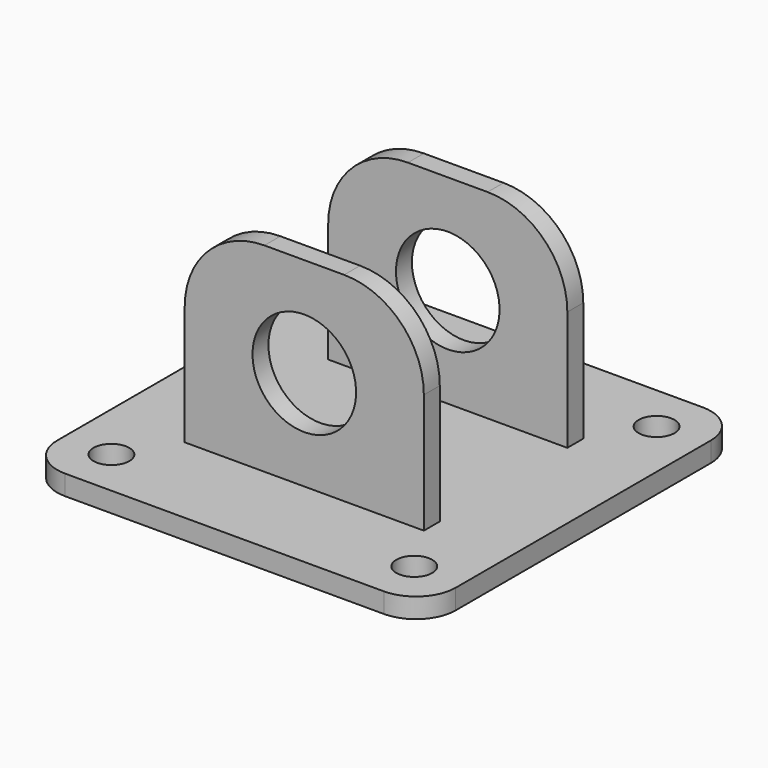
from build123d import *

# Parameters (mm, degrees)
F1_W     = 100
F1_H     = 100
F2_DEPTH = 5
F3_R     = 10
F5_D     = 9
F6_W     = 60
F6_H     = 5
F7_DEPTH = 50
F8_R     = 20
F10_D    = 26


# Not quite as in the source:
# - a pattern or mirror of a feature is missing from the dataset's text; its kind, count and spacing are read off the source's solid


with BuildPart() as f2:
    # F1 (on Top) → F2 (new body)
    with BuildSketch(Plane.XY):
        Rectangle(F1_W, F1_H)
    extrude(amount=F2_DEPTH)

    # F3
    f3_edges = [f2.edges().sort_by_distance(p)[0] for p in [
        (-50, 50, 2.5),
        (-50, -50, 2.5),
        (50, -50, 2.5),
        (50, 50, 2.5),
    ]]
    fillet(f3_edges, radius=F3_R)

    # F5 (through all)
    with Locations(Plane.XY.offset(5)):
        with Locations((-38, -38), (38, -38), (-38, -38), (38, 38)):
            f5 = Hole(F5_D / 2)

    # F5_copies: F5 across plane
    add(f5.mirror(Plane.ZX), mode=Mode.SUBTRACT)

    # F6 (on face) → F7 (join)
    with BuildSketch(Plane.XY.offset(5)):
        with Locations((0, -22.5)):
            Rectangle(F6_W, F6_H)
        with Locations((0, 22.5)):
            Rectangle(F6_W, F6_H)
    extrude(amount=F7_DEPTH)

    # F8
    f8_edges = [f2.edges().sort_by_distance(p)[0] for p in [
        (-30, -22.5, 55),
        (-30, 22.5, 55),
        (30, 22.5, 55),
        (30, -22.5, 55),
    ]]
    fillet(f8_edges, radius=F8_R)

    # F10 (through all)
    with Locations(Plane.XZ.offset(25)):
        with Locations((0, 30)):
            Hole(F10_D / 2)


solid = f2.part
